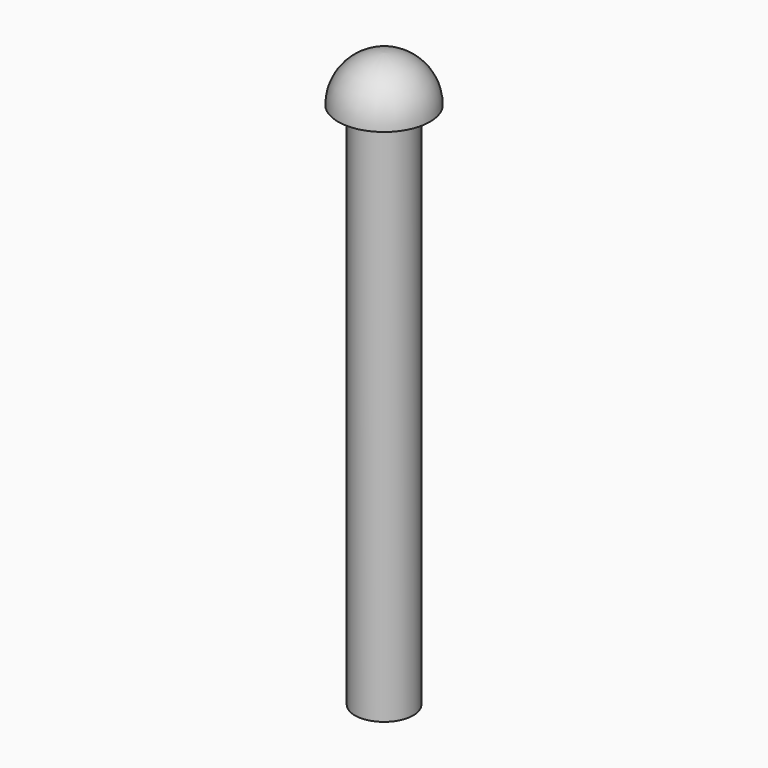
from build123d import *

# Parameters (mm, degrees)
F0_R     = 3.175
F1_DEPTH = 57.5
F2_R     = 5
F2_R_2   = 3.175
F3_DEPTH = 5
F4_R     = 4.99999


# Not quite as in the source:
# - a fillet or chamfer is up to 0.001 mm smaller than in the source, because OpenCascade refuses the exact size


with BuildPart() as f1:
    # F0 (on Top) → F1 (new body)
    with BuildSketch(Plane.XY):
        Circle(F0_R)
    extrude(amount=F1_DEPTH)

    # F2 (on face) → F3 (join)
    with BuildSketch(Plane.XY.offset(57.5)):
        Circle(F2_R)
        Circle(F2_R_2, mode=Mode.SUBTRACT)
        Circle(F2_R_2)
    extrude(amount=F3_DEPTH)

    # F4 (radius 5 in the source; OpenCascade refuses exactly that, so slightly less here)
    f4_edges = [f1.edges().sort_by_distance(p)[0] for p in [
        (-5, 0, 62.5),
    ]]
    fillet(f4_edges, radius=F4_R)


solid = f1.part
